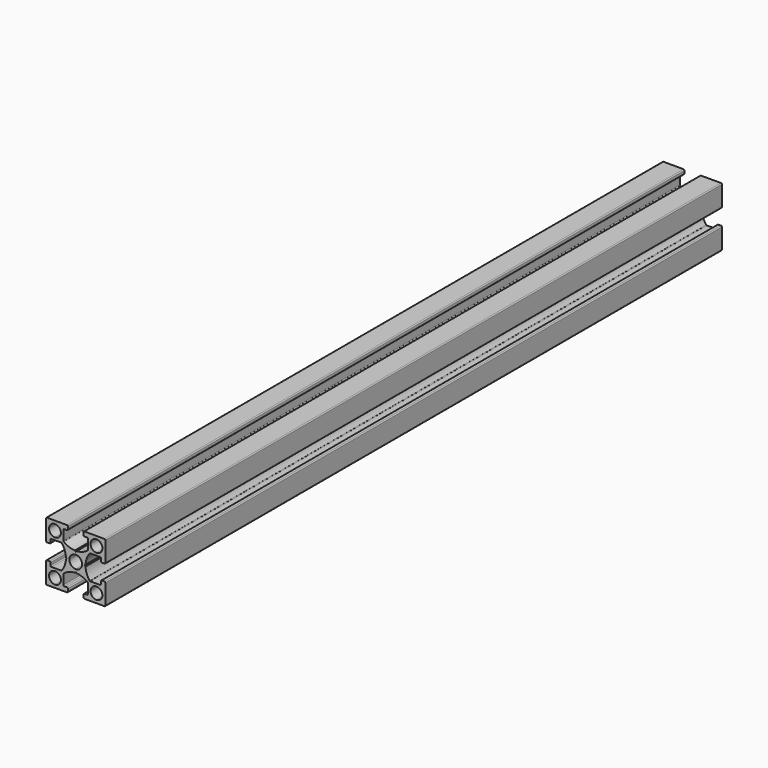
from build123d import *

# Parameters (mm, degrees)
F1_DEPTH = 260


# Not quite as in the source:
# - ends of sketch curves that miss each other by under 0.0002 mm in the source are joined


with BuildPart() as f1:
    # F0 (on Front) → F1 (new body)
    with BuildSketch(Plane.XZ):
        with BuildLine():
            ThreePointArc((-2.15, 0), (-1.5202795796, 1.5202795796), (0, 2.15))
            Line((0, 2.15), (0, 3))
            Line((0, 3), (-0.307277, 3.307278))
            ThreePointArc((-0.307277, 3.307278), (-2.2820211583, 3.7143800615), (-4.036565823, 4.7078182229))
            ThreePointArc((-4.036565823, 4.7078182229), (-4.1201572004, 4.8123081084), (-4.15, 4.94275))
            Line((-4.15, 4.94275), (-4.15, 8.2))
            ThreePointArc((-4.15, 8.2), (-4.0621320344, 8.4121320344), (-3.85, 8.5))
            Line((-3.85, 8.5), (-2.95, 8.5))
            ThreePointArc((-2.95, 8.5), (-2.7378679656, 8.5878679656), (-2.65, 8.8))
            Line((-2.65, 8.8), (-2.65, 9.7))
            ThreePointArc((-2.65, 9.7), (-2.7378679656, 9.9121320344), (-2.95, 10))
            Line((-2.95, 10), (-9.7, 10))
            ThreePointArc((-9.7, 10), (-9.9121320344, 9.9121320344), (-10, 9.7))
            Line((-10, 9.7), (-10, 2.95))
            ThreePointArc((-10, 2.95), (-9.9121320344, 2.7378679656), (-9.7, 2.65))
            Line((-9.7, 2.65), (-8.8, 2.65))
            ThreePointArc((-8.8, 2.65), (-8.5878679656, 2.7378679656), (-8.5, 2.95))
            Line((-8.5, 2.95), (-8.5, 3.85))
            ThreePointArc((-8.5, 3.85), (-8.4121320344, 4.0621320344), (-8.2, 4.15))
            Line((-8.2, 4.15), (-4.942749, 4.15))
            ThreePointArc((-4.942749, 4.15), (-4.812307461, 4.1201573706), (-4.7078173786, 4.0365666993))
            ThreePointArc((-4.7078173786, 4.0365666993), (-3.7143793747, 2.2820219924), (-3.3072773955, 0.3072779813))
            Line((-3.3072773955, 0.3072779813), (-3, 0))
            Line((-3, 0), (-2.15, 0))
        make_face()
        with BuildLine():
            ThreePointArc((-7, 5), (-8.4142135624, 5.5857864376), (-9, 7))
            ThreePointArc((-9, 7), (-8.4142135624, 8.4142135624), (-7, 9))
            ThreePointArc((-7, 9), (-5.5857864376, 8.4142135624), (-5, 7))
            ThreePointArc((-5, 7), (-5.5857864376, 5.5857864376), (-7, 5))
        make_face(mode=Mode.SUBTRACT)
        with BuildLine():
            ThreePointArc((0, 2.15), (1.5202795796, 1.5202795796), (2.15, 0))
            Line((2.15, 0), (3, 0))
            Line((3, 0), (3.307278, 0.307278))
            ThreePointArc((3.307278, 0.307278), (3.7143803747, 2.2820219924), (4.7078187099, 4.0365664363))
            ThreePointArc((4.7078187099, 4.0365664363), (4.812308461, 4.1201573706), (4.94275, 4.15))
            Line((4.94275, 4.15), (8.2, 4.15))
            ThreePointArc((8.2, 4.15), (8.4121320344, 4.0621320344), (8.5, 3.85))
            Line((8.5, 3.85), (8.5, 2.95))
            ThreePointArc((8.5, 2.95), (8.5878679656, 2.7378679656), (8.8, 2.65))
            Line((8.8, 2.65), (9.7, 2.65))
            ThreePointArc((9.7, 2.65), (9.9121320344, 2.7378679656), (10, 2.95))
            Line((10, 2.95), (10, 9.7))
            ThreePointArc((10, 9.7), (9.9121320344, 9.9121320344), (9.7, 10))
            Line((9.7, 10), (2.95, 10))
            ThreePointArc((2.95, 10), (2.7378679656, 9.9121320344), (2.65, 9.7))
            Line((2.65, 9.7), (2.65, 8.8))
            ThreePointArc((2.65, 8.8), (2.7378679656, 8.5878679656), (2.95, 8.5))
            Line((2.95, 8.5), (3.85, 8.5))
            ThreePointArc((3.85, 8.5), (4.0621320344, 8.4121320344), (4.15, 8.2))
            Line((4.15, 8.2), (4.15, 4.94275))
            ThreePointArc((4.15, 4.94275), (4.1201572004, 4.8123081084), (4.036566086, 4.7078178916))
            ThreePointArc((4.036566086, 4.7078178916), (2.2820216259, 3.7143802371), (0.3072779813, 3.3072783955))
            Line((0.3072779813, 3.3072783955), (0, 3))
            Line((0, 3), (0, 2.15))
        make_face()
        with BuildLine():
            ThreePointArc((7, 9), (8.4142135624, 8.4142135624), (9, 7))
            ThreePointArc((9, 7), (8.4142135624, 5.5857864376), (7, 5))
            ThreePointArc((7, 5), (5.5857864376, 5.5857864376), (5, 7))
            ThreePointArc((5, 7), (5.5857864376, 8.4142135624), (7, 9))
        make_face(mode=Mode.SUBTRACT)
        with BuildLine():
            Line((3, 0), (2.15, 0))
            ThreePointArc((2.15, 0), (1.5202795796, -1.5202795796), (0, -2.15))
            Line((0, -2.15), (0, -3))
            Line((0, -3), (0.307278, -3.307277))
            ThreePointArc((0.307278, -3.307277), (2.2820216259, -3.7143792371), (4.036565823, -4.7078172229))
            ThreePointArc((4.036565823, -4.7078172229), (4.1201572004, -4.8123071084), (4.15, -4.942749))
            Line((4.15, -4.942749), (4.15, -8.2))
            ThreePointArc((4.15, -8.2), (4.0621320344, -8.4121320344), (3.85, -8.5))
            Line((3.85, -8.5), (2.95, -8.5))
            ThreePointArc((2.95, -8.5), (2.7378679656, -8.5878679656), (2.65, -8.8))
            Line((2.65, -8.8), (2.65, -9.7))
            ThreePointArc((2.65, -9.7), (2.7378679656, -9.9121320344), (2.95, -10))
            Line((2.95, -10), (9.7, -10))
            ThreePointArc((9.7, -10), (9.9121320344, -9.9121320344), (10, -9.7))
            Line((10, -9.7), (10, -2.95))
            ThreePointArc((10, -2.95), (9.9121320344, -2.7378679656), (9.7, -2.65))
            Line((9.7, -2.65), (8.8, -2.65))
            ThreePointArc((8.8, -2.65), (8.5878679656, -2.7378679656), (8.5, -2.95))
            Line((8.5, -2.95), (8.5, -3.85))
            ThreePointArc((8.5, -3.85), (8.4121320344, -4.0621320344), (8.2, -4.15))
            Line((8.2, -4.15), (4.94275, -4.15))
            ThreePointArc((4.94275, -4.15), (4.8123081084, -4.1201572004), (4.7078178916, -4.036566086))
            ThreePointArc((4.7078178916, -4.036566086), (3.7143800615, -2.2820211583), (3.3072783483, -0.3072769835))
            Line((3.3072783483, -0.3072769835), (3, 0))
        make_face()
        with BuildLine():
            ThreePointArc((7, -5), (8.4142135624, -5.5857864376), (9, -7))
            ThreePointArc((9, -7), (8.4142135624, -8.4142135624), (7, -9))
            ThreePointArc((7, -9), (5.5857864376, -8.4142135624), (5, -7))
            ThreePointArc((5, -7), (5.5857864376, -5.5857864376), (7, -5))
        make_face(mode=Mode.SUBTRACT)
        with BuildLine():
            Line((0, -3), (0, -2.15))
            ThreePointArc((0, -2.15), (-1.5202795796, -1.5202795796), (-2.15, 0))
            Line((-2.15, 0), (-3, 0))
            Line((-3, 0), (-3.307277, -0.307277))
            ThreePointArc((-3.307277, -0.307277), (-3.7143790615, -2.2820211583), (-4.7078172229, -4.036565823))
            ThreePointArc((-4.7078172229, -4.036565823), (-4.8123071084, -4.1201572004), (-4.942749, -4.15))
            Line((-4.942749, -4.15), (-8.2, -4.15))
            ThreePointArc((-8.2, -4.15), (-8.4121320344, -4.0621320344), (-8.5, -3.85))
            Line((-8.5, -3.85), (-8.5, -2.95))
            ThreePointArc((-8.5, -2.95), (-8.5878679656, -2.7378679656), (-8.8, -2.65))
            Line((-8.8, -2.65), (-9.7, -2.65))
            ThreePointArc((-9.7, -2.65), (-9.9121320344, -2.7378679656), (-10, -2.95))
            Line((-10, -2.95), (-10, -9.7))
            ThreePointArc((-10, -9.7), (-9.9121320344, -9.9121320344), (-9.7, -10))
            Line((-9.7, -10), (-2.95, -10))
            ThreePointArc((-2.95, -10), (-2.7378679656, -9.9121320344), (-2.65, -9.7))
            Line((-2.65, -9.7), (-2.65, -8.8))
            ThreePointArc((-2.65, -8.8), (-2.7378679656, -8.5878679656), (-2.95, -8.5))
            Line((-2.95, -8.5), (-3.85, -8.5))
            ThreePointArc((-3.85, -8.5), (-4.0621320344, -8.4121320344), (-4.15, -8.2))
            Line((-4.15, -8.2), (-4.15, -4.942749))
            ThreePointArc((-4.15, -4.942749), (-4.1201572004, -4.8123071084), (-4.036566086, -4.7078168916))
            ThreePointArc((-4.036566086, -4.7078168916), (-2.2820211583, -3.7143790615), (-0.3072769835, -3.3072773483))
            Line((-0.3072769835, -3.3072773483), (0, -3))
        make_face()
        with BuildLine():
            ThreePointArc((-7, -9), (-8.4142135624, -8.4142135624), (-9, -7))
            ThreePointArc((-9, -7), (-8.4142135624, -5.5857864376), (-7, -5))
            ThreePointArc((-7, -5), (-5.5857864376, -5.5857864376), (-5, -7))
            ThreePointArc((-5, -7), (-5.5857864376, -8.4142135624), (-7, -9))
        make_face(mode=Mode.SUBTRACT)
    extrude(amount=F1_DEPTH)


solid = f1.part
